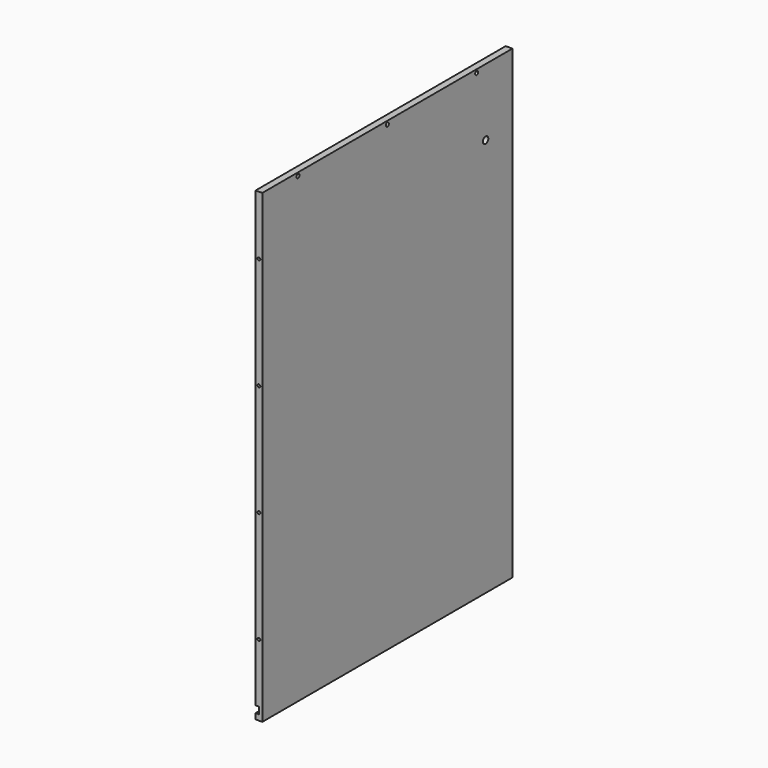
from build123d import *

# Parameters (mm, degrees)
F0_W      = 280
F0_H      = 417
F1_DEPTH  = 6
F3_D      = 3.4
F4_W      = 280
F4_H      = 6.1
F5_DEPTH  = 3
F8_D      = 2.5
F8_DEPTH  = 16.5
F8_TIP    = 0.7510757738
F9_D      = 6
F10_D     = 2.5
F10_DEPTH = 16.5
F10_TIP   = 0.7510757738


# Not quite as in the source:
# - a feature names something its author has since deleted; it is built from what else it names


with BuildPart() as f1:
    # F0 (on Right) → F1 (new body)
    with BuildSketch(Plane.YZ):
        Rectangle(F0_W, F0_H)
    extrude(amount=F1_DEPTH)

    # F3 (through all)
    with Locations(Plane.YZ.offset(6)):
        with Locations((100, 205.5), (0, 205.5), (-100, 205.5)):
            Hole(F3_D / 2)


with BuildPart() as f5:
    # F4 (on face) → F5 (new body)
    with BuildSketch(Plane(origin=(0, 0, 0), x_dir=(0, -1, 0), z_dir=(-1, 0, 0))):
        with Locations((0, -200.45)):
            Rectangle(F4_W, F4_H)
    extrude(amount=-F5_DEPTH)


with BuildPart() as f1_1:
    add(f1.part)

    # F6: cut F5
    add(f5.part, mode=Mode.SUBTRACT)

    # F8
    with Locations(Plane.XZ.offset(140)):
        with Locations((3, 155.5), (3, 55.5), (3, -44.5)):
            Hole(F8_D / 2, depth=F8_DEPTH)
            with Locations((0, 0, -(F8_DEPTH + F8_TIP / 2))):  # 118° drill point
                Cone(0, F8_D / 2, F8_TIP, mode=Mode.SUBTRACT)

    # F9 (through all)
    with Locations(Plane.YZ.offset(6)):
        with Locations((110, 148.5)):
            Hole(F9_D / 2)

    # F10
    with Locations(Plane.XZ.offset(140)):
        with Locations((3, -144.5)):
            Hole(F10_D / 2, depth=F10_DEPTH)
            with Locations((0, 0, -(F10_DEPTH + F10_TIP / 2))):  # 118° drill point
                Cone(0, F10_D / 2, F10_TIP, mode=Mode.SUBTRACT)


solid = f1_1.part
